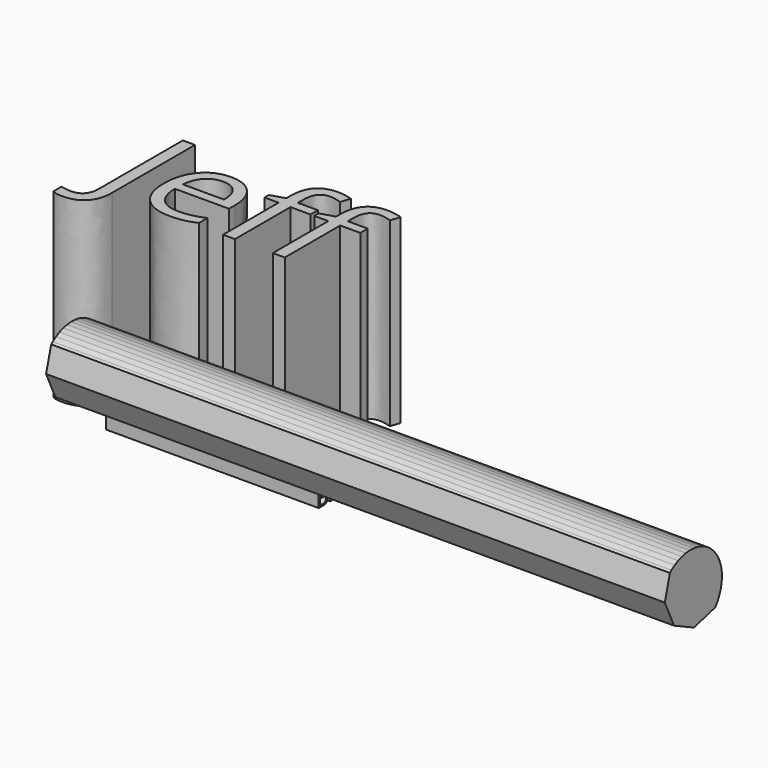
from build123d import *

# Parameters (mm, degrees)
F1_DEPTH     = 2514.6
F2_TEXT_SIZE = 596.9739415579
F3_DEPTH     = 736.6
F4_TEXT_SIZE = 92.911389139
F5_DEPTH     = 863.6


# Not quite as in the source:
# - Text() gives the source's letters only with a copy of the font that has no kerning and outlines rounded to 1/6400 em; it was checked with that copy


with BuildPart() as f1:
    # F0 (on Right) → F1 (new body)
    with BuildSketch(Plane.YZ):
        Polygon((-873.756865057, 556.2420334241), (-881.4057266782, 549.5067879491), (-907.4715634694, 454.410344719), (-860.6274658142, 352.4315819947), (-759.1921199822, 304.4221230532), (-650.6282516164, 332.8461272991), (-639.3861989363, 349.3670239129), (-630.3034105933, 367.1666511367), (-623.5231275856, 385.9642982161), (-619.1522790264, 405.4635150275), (-617.2597958085, 425.3567872736), (-617.8755235228, 445.3303861674), (-620.9897517755, 465.0693161226), (-626.5533673266, 484.2622824224), (-634.4786286354, 502.606600523), (-644.6405495967, 519.8129695695), (-656.8788706464, 535.6100348434), (-671.0005861509, 549.7486671888), (-686.7829882208, 562.0058919275), (-703.9771789473, 572.1884053032), (-722.3119956715, 580.1356229973), (-741.4982873809, 585.7222126393), (-761.233474794, 588.8600703733), (-781.2063222159, 589.4997103083), (-801.1018459117, 587.6310449406), (-820.6062815877, 583.2835442391), (-839.4120326418, 576.5257708872), (-857.222521146, 567.4642990073), align=None)
    extrude(amount=F1_DEPTH)


with BuildPart() as f3:
    # F2 (on Top) → F3 (new body)
    with BuildSketch(Plane.XY):
        with Locations((-380.6257545948, -232.501193881)):
            Text('Jeff', F2_TEXT_SIZE, font='Open Sans', text_align=(TextAlign.LEFT, TextAlign.BOTTOM))
    extrude(amount=F3_DEPTH)


with BuildPart() as f5:
    # F4 (on Right) → F5 (new body)
    with BuildSketch(Plane.YZ):
        with Locations((-611.0147237778, 130.9559494257)):
            Text('Bruh', F4_TEXT_SIZE, font='Open Sans', text_align=(TextAlign.LEFT, TextAlign.BOTTOM))
    extrude(amount=F5_DEPTH)


solid = Compound([f1.part, f3.part, f5.part])
